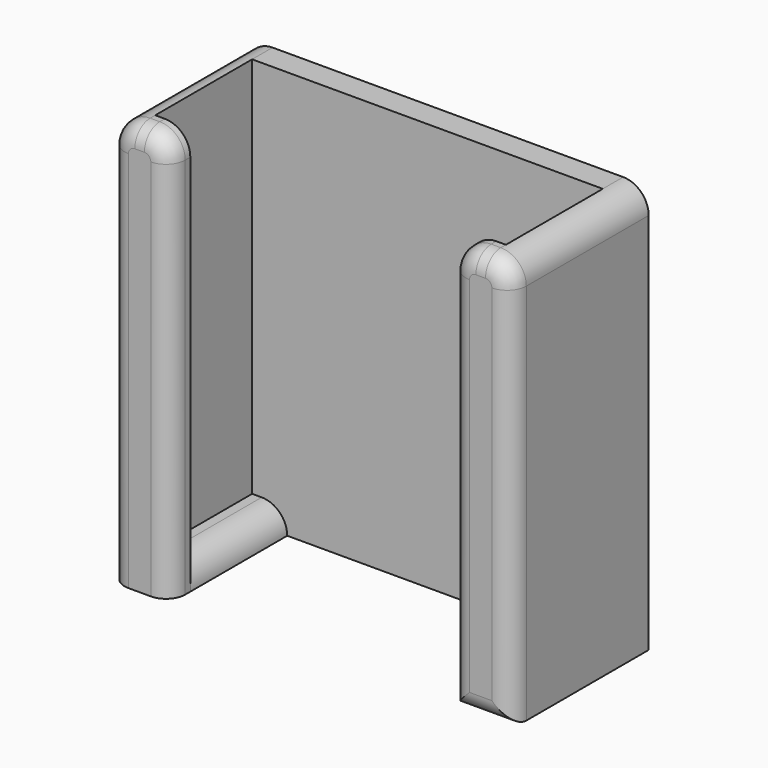
from build123d import *

# Parameters (mm, degrees)
F0_W     = 63
F0_H     = 27
F0_W_2   = 55
F0_H_2   = 19
F1_DEPTH = 60
F2_DEPTH = 4
F3_W     = 44
F3_H     = 64
F4_DEPTH = 23
F5_R     = 3.99999
F6_R     = 3


# Not quite as in the source:
# - a fillet or chamfer is up to 0.001 mm smaller than in the source, because OpenCascade refuses the exact size


with BuildPart() as f1:
    # F0 (on Top) → F1 (new body)
    with BuildSketch(Plane.XY):
        Rectangle(F0_W, F0_H)
        Rectangle(F0_W_2, F0_H_2, mode=Mode.SUBTRACT)
    extrude(amount=F1_DEPTH)

    # F0 (on Top) → F2 (join)
    with BuildSketch(Plane.XY):
        Rectangle(F0_W, F0_H)
        Rectangle(F0_W_2, F0_H_2, mode=Mode.SUBTRACT)
        Rectangle(F0_W_2, F0_H_2)
    extrude(amount=-F2_DEPTH)

    # F3 (on face) → F4 (cut)
    with BuildSketch(Plane.XZ.offset(13.5)):
        with Locations((0, 28)):
            Rectangle(F3_W, F3_H)
    extrude(amount=-F4_DEPTH, mode=Mode.SUBTRACT)

    # F5 (radius 4 in the source; OpenCascade refuses exactly that, so slightly less here)
    f5_edges = [f1.edges().sort_by_distance(p)[0] for p in [
        (-22, -11.5, 60),
        (-22, 0, 0),
        (22, 0, 0),
        (-31.5, 0, 60),
        (31.5, 0, 60),
        (22, -11.5, 60),
    ]]
    fillet(f5_edges, radius=F5_R)

    # F6
    f6_edges = [f1.edges().sort_by_distance(p)[0] for p in [
        (-22, -13.5, 26.000005),
        (22, -13.5, 26.000005),
        (23.17157, -13.5, 58.82843),
        (26.75, -13.5, -4),
        (26.75, -13.5, 60),
        (31.5, -13.5, 26.000005),
        (30.32843, -13.5, 58.82843),
    ]]
    fillet(f6_edges, radius=F6_R)


solid = f1.part
